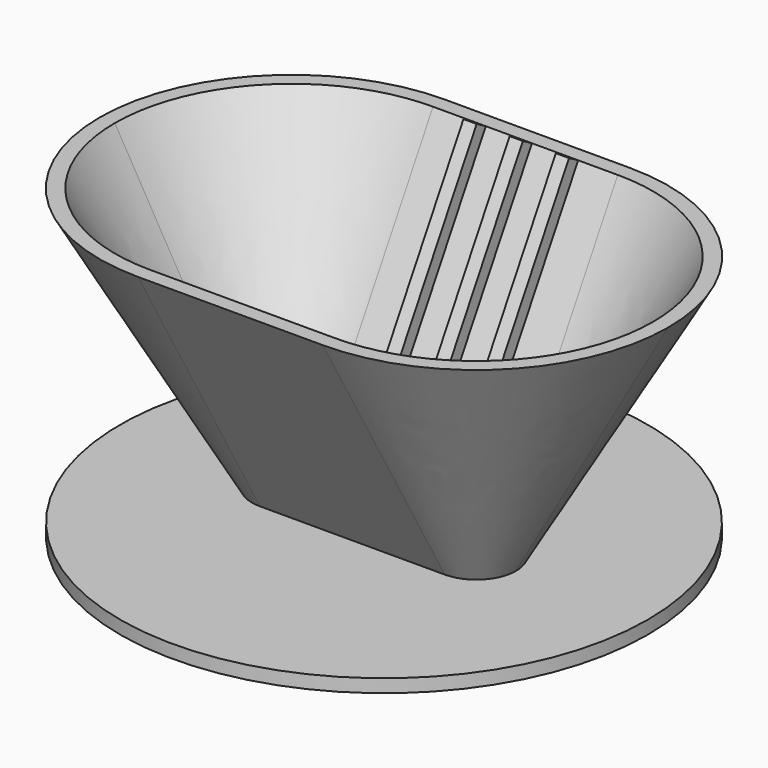
from build123d import *

# Parameters (mm, degrees)
F1_DEPTH  = 50
F1_TAPER  = -30
F2_T      = -2.5
F3_R      = 50
F4_DEPTH  = 2.5
F5_R      = 27.5
F5_R_2    = 25
F6_DEPTH  = 10
F7_R      = 2.5
F8_DEPTH  = 15.001
F9_SIZE   = 1
F10_W     = 2.5
F10_H     = 54.848275
F11_DEPTH = 2.5


with BuildPart() as f1:
    # F0 (on Top) → F1 (new body)
    with BuildSketch(Plane.XY):
        with BuildLine():
            ThreePointArc((25, 0), (22.803301, 5.303301), (17.5, 7.5))
            Line((17.5, 7.5), (-17.5, 7.5))
            ThreePointArc((-17.5, 7.5), (-22.803301, 5.303301), (-25, 0))
            ThreePointArc((-25, 0), (-22.803301, -5.303301), (-17.5, -7.5))
            Line((-17.5, -7.5), (17.5, -7.5))
            ThreePointArc((17.5, -7.5), (22.803301, -5.303301), (25, 0))
        make_face()
    extrude(amount=F1_DEPTH, taper=F1_TAPER)

    # F2
    f2_openings = [f1.faces().sort_by_distance(p)[0] for p in [
        (0, 0, 50),
    ]]
    offset(amount=F2_T, openings=f2_openings)

    # F3 (on face) → F4 (join)
    with BuildSketch(Plane(origin=(0, 0, 0), x_dir=(1, 0, 0), z_dir=(0, 0, -1))):
        Circle(F3_R)
    extrude(amount=F4_DEPTH)

    # F5 (on face) → F6 (join)
    with BuildSketch(Plane(origin=(0, 0, -2.5), x_dir=(1, 0, 0), z_dir=(0, 0, -1))):
        Circle(F5_R)
        Circle(F5_R_2, mode=Mode.SUBTRACT)
    extrude(amount=F6_DEPTH)

    # F7 (on face) → F8 (cut, through all)
    with BuildSketch(Plane.XY.offset(2.5)):
        with Locations((-17.5, 0)):
            Circle(F7_R)
        with Locations((-8.75, 0)):
            Circle(F7_R)
        Circle(F7_R)
        with Locations((8.75, 0)):
            Circle(F7_R)
        with Locations((17.5, 0)):
            Circle(F7_R)
    extrude(amount=-F8_DEPTH, mode=Mode.SUBTRACT)

    # F9
    f9_edges = [f1.edges().sort_by_distance(p)[0] for p in [
        (-20, 0, 2.5),
        (-11.25, 0, 2.5),
        (-2.5, 0, 2.5),
        (6.25, 0, 2.5),
        (15, 0, 2.5),
    ]]
    chamfer(f9_edges, length=F9_SIZE)

    # F10 (on face) → F11 (join)
    with BuildSketch(Plane(origin=(0, 3.459936, -1.997595), x_dir=(1, 0, 0), z_dir=(0, -0.866025, 0.5))):
        with Locations((0, 32.617513)):
            Rectangle(F10_W, F10_H)
        with Locations((-8.75, 32.617513)):
            Rectangle(F10_W, F10_H)
        with Locations((8.75, 32.617513)):
            Rectangle(F10_W, F10_H)
    extrude(amount=F11_DEPTH)


solid = f1.part
